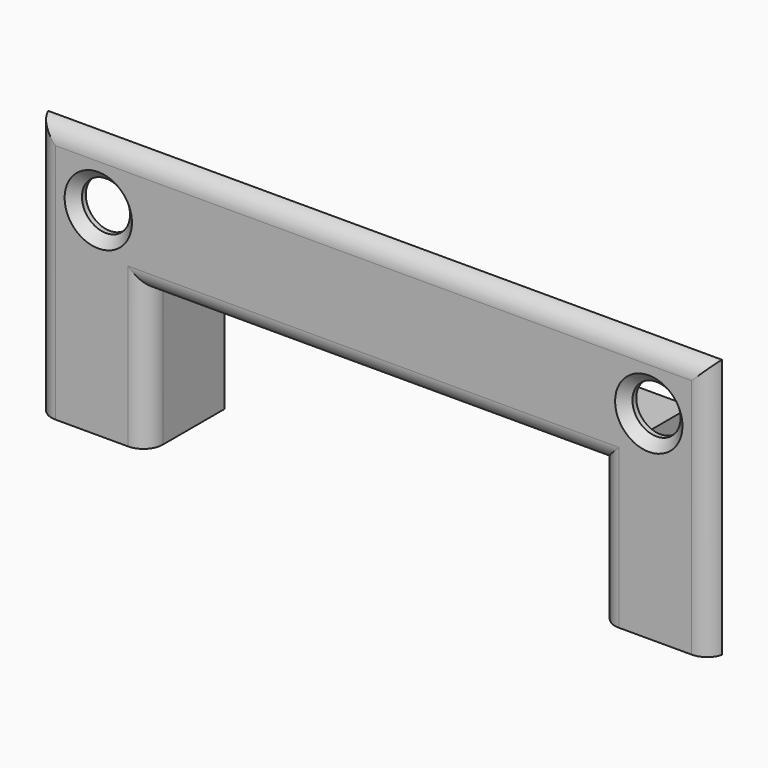
from build123d import *

# Parameters (mm, degrees)
F1_DEPTH       = 1.5
F2_DEPTH       = 10
F3_D           = 5
F3_CSINK_D     = 7
F3_CSINK_ANGLE = 90
F4_T1_DEPTH    = 36.6824583655
F4_T3_DEPTH    = 79.6824583655
F4_T5_DEPTH    = 19.5
F4_T7_DEPTH    = 47
F4_T13_DEPTH   = 52
F4_T17_DEPTH   = 24.5
F4_T24_DEPTH   = 24.5
F4_T28_DEPTH   = 52
F5_R           = 1


# Not quite as in the source:
# - a fillet or chamfer that OpenCascade refuses, or shapes differently, is made with other operations: its cross-section is extruded or revolved along the edge and cut away or added


with BuildPart() as f1:
    # F0 (on Front) → F1 (new body)
    with BuildSketch(Plane.XZ):
        Polygon((35, 27), (-35, 27), (-35, 0), (-25, 0), (-25, 16), (25, 16), (25, 0), (35, 0), align=None)
        Polygon((-25, 16), (-25, 0), (-23.5, 0), (-23.5, 14.5), (23.5, 14.5), (23.5, 0), (25, 0), (25, 16), align=None)
    extrude(amount=-F1_DEPTH)

    # F0 (on Front) → F2 (join)
    with BuildSketch(Plane.XZ):
        Polygon((-25, 16), (-25, 0), (-23.5, 0), (-23.5, 14.5), (23.5, 14.5), (23.5, 0), (25, 0), (25, 16), align=None)
    extrude(amount=-F2_DEPTH)

    # F3 (through all)
    with Locations(Plane.XZ):
        with Locations((28.6, 20.6), (-28.6, 20.6)):
            CounterSinkHole(F3_D / 2, F3_CSINK_D / 2, counter_sink_angle=F3_CSINK_ANGLE)

    # F4: fillet of radius 2 on 6 edges, made by hand

    # F4_s2 → F4_t1 (cut)
    with BuildSketch(Plane.XY.offset(-4.8412291828)):
        with BuildLine():
            ThreePointArc((-33.0635083269, 0), (-34.2882531983, 0.4188611699), (-35, 1.5))
            Line((-35, 1.5), (-35.0387298335, 1.49))
            ThreePointArc((-35.0387298335, 1.49), (-35.04, 0.75), (-35.04, 0))
            Line((-35.04, 0), (-35, -0.04))
            Line((-35, -0.04), (-33.0635083269, -0.04))
            Line((-33.0635083269, -0.04), (-33.0635083269, 0))
        make_face()
        with BuildLine():
            ThreePointArc((35, 1.5), (34.2882531983, 0.4188611699), (33.0635083269, 0))
            Line((33.0635083269, 0), (33.0635083269, -0.04))
            Line((33.0635083269, -0.04), (35, -0.04))
            Line((35, -0.04), (35.04, 0))
            ThreePointArc((35.04, 0), (35.04, 0.75), (35.0387298335, 1.49))
            Line((35.0387298335, 1.49), (35, 1.5))
        make_face()
    extrude(amount=F4_T1_DEPTH, mode=Mode.SUBTRACT)

    # F4_s4 → F4_t3 (cut)
    with BuildSketch(Plane.YZ.offset(-39.8412291828)):
        with BuildLine():
            ThreePointArc((1.5, 27), (0.4188611699, 26.2882531983), (0, 25.0635083269))
            Line((0, 25.0635083269), (-0.04, 25.0635083269))
            Line((-0.04, 25.0635083269), (-0.04, 27))
            Line((-0.04, 27), (0, 27.04))
            ThreePointArc((0, 27.04), (0.75, 27.04), (1.49, 27.0387298335))
            Line((1.49, 27.0387298335), (1.5, 27))
        make_face()
    extrude(amount=F4_T3_DEPTH, mode=Mode.SUBTRACT)

    # F4_s6 → F4_t5 (cut)
    with BuildSketch(Plane.XY.offset(-5)):
        with BuildLine():
            ThreePointArc((-25.5, 0), (-24.0857864376, 0.5857864376), (-23.5, 2))
            Line((-23.5, 2), (-23.46, 2))
            Line((-23.46, 2), (-23.46, -0.04))
            Line((-23.46, -0.04), (-25.5, -0.04))
            Line((-25.5, -0.04), (-25.5, 0))
        make_face()
        with BuildLine():
            ThreePointArc((25.5, 0), (24.0857864376, 0.5857864376), (23.5, 2))
            Line((23.5, 2), (23.46, 2))
            Line((23.46, 2), (23.46, -0.04))
            Line((23.46, -0.04), (25.5, -0.04))
            Line((25.5, -0.04), (25.5, 0))
        make_face()
    extrude(amount=F4_T5_DEPTH, mode=Mode.SUBTRACT)

    # F4_s8 → F4_t7 (cut)
    with BuildSketch(Plane.YZ.offset(-23.5)):
        with BuildLine():
            ThreePointArc((0, 16.5), (0.5857864376, 15.0857864376), (2, 14.5))
            Line((2, 14.5), (2, 14.46))
            Line((2, 14.46), (-0.04, 14.46))
            Line((-0.04, 14.46), (-0.04, 16.5))
            Line((-0.04, 16.5), (0, 16.5))
        make_face()
    extrude(amount=F4_T7_DEPTH, mode=Mode.SUBTRACT)


with BuildPart() as f4_tool11:
    # F4_s12 → F4_t13 (new body)
    with BuildSketch(Plane.YZ.offset(-28.5)):
        with BuildLine():
            ThreePointArc((0, 16.5), (0.5857864376, 15.0857864376), (2, 14.5))
            Line((2, 14.5), (2, 14.46))
            Line((2, 14.46), (-0.04, 14.46))
            Line((-0.04, 14.46), (-0.04, 16.5))
            Line((-0.04, 16.5), (0, 16.5))
        make_face()
    extrude(amount=F4_T13_DEPTH)

    split(bisect_by=Plane.YZ.offset(-23.5), keep=Keep.BOTTOM)


with BuildPart() as f4_tool15:
    # F4_s16 → F4_t17 (new body)
    with BuildSketch(Plane.XY.offset(-5)):
        with BuildLine():
            ThreePointArc((-25.5, 0), (-24.0857864376, 0.5857864376), (-23.5, 2))
            Line((-23.5, 2), (-23.46, 2))
            Line((-23.46, 2), (-23.46, -0.04))
            Line((-23.46, -0.04), (-25.5, -0.04))
            Line((-25.5, -0.04), (-25.5, 0))
        make_face()
    extrude(amount=F4_T17_DEPTH)

    split(bisect_by=Plane.XY.offset(14.5), keep=Keep.TOP)


with BuildPart() as f4_tool11_1:
    add(f4_tool11.part)

    # F4_t19: intersect F4_tool15
    add(f4_tool15.part, mode=Mode.INTERSECT)


with BuildPart() as f1_1:
    add(f1.part)

    # F4_t9: cut F4_tool11
    add(f4_tool11_1.part, mode=Mode.SUBTRACT)


with BuildPart() as f4_tool22:
    # F4_s23 → F4_t24 (new body)
    with BuildSketch(Plane.XY.offset(19.5)):
        with BuildLine():
            ThreePointArc((25.5, 0), (24.0857864376, 0.5857864376), (23.5, 2))
            Line((23.5, 2), (23.46, 2))
            Line((23.46, 2), (23.46, -0.04))
            Line((23.46, -0.04), (25.5, -0.04))
            Line((25.5, -0.04), (25.5, 0))
        make_face()
    extrude(amount=-F4_T24_DEPTH)

    split(bisect_by=Plane.XY.offset(14.5), keep=Keep.TOP)


with BuildPart() as f4_tool26:
    # F4_s27 → F4_t28 (new body)
    with BuildSketch(Plane.YZ.offset(-23.5)):
        with BuildLine():
            ThreePointArc((0, 16.5), (0.5857864376, 15.0857864376), (2, 14.5))
            Line((2, 14.5), (2, 14.46))
            Line((2, 14.46), (-0.04, 14.46))
            Line((-0.04, 14.46), (-0.04, 16.5))
            Line((-0.04, 16.5), (0, 16.5))
        make_face()
    extrude(amount=F4_T28_DEPTH)

    split(bisect_by=Plane.YZ.offset(23.5), keep=Keep.TOP)


with BuildPart() as f4_tool22_1:
    add(f4_tool22.part)

    # F4_t30: intersect F4_tool26
    add(f4_tool26.part, mode=Mode.INTERSECT)


with BuildPart() as f1_2:
    add(f1_1.part)

    # F4_t20: cut F4_tool22
    add(f4_tool22_1.part, mode=Mode.SUBTRACT)

    # F5
    f5_edges = [f1_2.edges().sort_by_distance(p)[0] for p in [
        (25, 1.5, 8),
        (0, 1.5, 16),
        (-25, 1.5, 8),
    ]]
    fillet(f5_edges, radius=F5_R)


solid = f1_2.part
